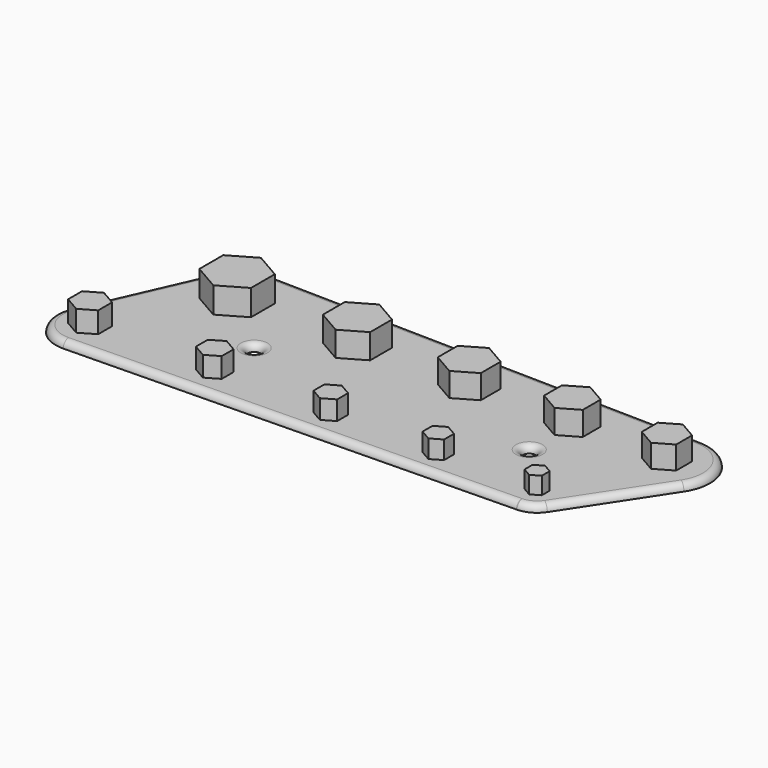
from build123d import *

# Parameters (mm, degrees)
F1_DEPTH  = 6.35
F2_DEPTH  = 3.175
F3_DEPTH  = 2.8222222222
F4_DEPTH  = 2.4694444444
F5_DEPTH  = 2.4694444444
F6_DEPTH  = 2.1166666667
F7_DEPTH  = 1.4111111111
F8_DEPTH  = 1.0583333333
F9_DEPTH  = 0.3527777778
F10_DEPTH = 0.7055555556
F12_DEPTH = 2.54
F13_R     = 2.38125
F14_DEPTH = 25.4
F15_R     = 2.53999
F16_R     = 2.53999
F18_DEPTH = 2.54


# Not quite as in the source:
# - a fillet or chamfer is up to 0.001 mm smaller than in the source, because OpenCascade refuses the exact size


with BuildPart() as f1:
    # F0 (on Top) → F1 (new body)
    with BuildSketch(Plane.XY):
        Polygon((152.4, 3.6661742094), (152.4, 0), (152.4, -3.6661742094), (158.75, -7.3323484187), (165.1, -3.6661742094), (165.1, 3.6661742094), (158.75, 7.3323484187), align=None)
    extrude(amount=F1_DEPTH)

    # F6 (add): a face of the model
    f6_faces = [f1.faces().sort_by_distance(p)[0] for p in [
        (158.75, 0, 6.35),
    ]]
    extrude(f6_faces, amount=F6_DEPTH)


with BuildPart() as f1b:
    # F0 (on Top) → F1, piece 2 (new body)
    with BuildSketch(Plane.XY):
        Polygon((144.4625, -36.2669128953), (141.2875, -34.4338257906), (138.1125, -36.2669128953), (138.1125, -39.9330871047), (141.2875, -41.7661742094), (144.4625, -39.9330871047), align=None)
    extrude(amount=F1_DEPTH)


with BuildPart() as f1c:
    # F0 (on Top) → F1, piece 3 (new body)
    with BuildSketch(Plane.XY):
        Polygon((116.68125, 4.1244459855), (116.68125, 0), (123.825, 0), (130.96875, 0), (130.96875, 4.1244459855), (123.825, 8.248891971), align=None)
        Polygon((123.825, 0), (116.68125, 0), (116.68125, -4.1244459855), (123.825, -8.248891971), (130.96875, -4.1244459855), (130.96875, 0), align=None)
    extrude(amount=F1_DEPTH)

    # F5 (add): a face of the model
    f5_faces = [f1c.faces().sort_by_distance(p)[0] for p in [
        (123.825, 0, 6.35),
    ]]
    extrude(f5_faces, amount=F5_DEPTH)


with BuildPart() as f1d:
    # F0 (on Top) → F1, piece 4 (new body)
    with BuildSketch(Plane.XY):
        Polygon((108.74375, -35.8086411192), (104.775, -33.5172822383), (100.80625, -35.8086411192), (100.80625, -40.3913588808), (104.775, -42.6827177617), (108.74375, -40.3913588808), align=None)
    extrude(amount=F1_DEPTH)

    # F9 (add): a face of the model
    f9_faces = [f1d.faces().sort_by_distance(p)[0] for p in [
        (104.775, -38.1, 6.35),
    ]]
    extrude(f9_faces, amount=F9_DEPTH)


with BuildPart() as f1e:
    # F0 (on Top) → F1, piece 5 (new body)
    with BuildSketch(Plane.XY):
        Polygon((77.7875, 4.5827177617), (77.7875, 0), (85.725, 0), (93.6625, 0), (93.6625, 4.5827177617), (85.725, 9.1654355234), align=None)
        Polygon((85.725, 0), (77.7875, 0), (77.7875, -4.5827177617), (85.725, -9.1654355234), (93.6625, -4.5827177617), (93.6625, 0), align=None)
    extrude(amount=F1_DEPTH)

    # F4 (add): a face of the model
    f4_faces = [f1e.faces().sort_by_distance(p)[0] for p in [
        (85.725, 0, 6.35),
    ]]
    extrude(f4_faces, amount=F4_DEPTH)


with BuildPart() as f1f:
    # F0 (on Top) → F1, piece 6 (new body)
    with BuildSketch(Plane.XY):
        Polygon((69.453125, -35.5795052311), (65.0875, -33.0590104621), (60.721875, -35.5795052311), (60.721875, -40.6204947689), (65.0875, -43.1409895379), (69.453125, -40.6204947689), align=None)
    extrude(amount=F1_DEPTH)

    # F10 (add): a face of the model
    f10_faces = [f1f.faces().sort_by_distance(p)[0] for p in [
        (65.0875, -38.1, 6.35),
    ]]
    extrude(f10_faces, amount=F10_DEPTH)


with BuildPart() as f1g:
    # F0 (on Top) → F1, piece 7 (new body)
    with BuildSketch(Plane.XY):
        Polygon((35.71875, 5.0409895379), (35.71875, 0), (44.45, 0), (53.18125, 0), (53.18125, 5.0409895379), (44.45, 10.0819790757), align=None)
        Polygon((44.45, 0), (35.71875, 0), (35.71875, -5.0409895379), (44.45, -10.0819790757), (53.18125, -5.0409895379), (53.18125, 0), align=None)
    extrude(amount=F1_DEPTH)

    # F3 (add): a face of the model
    f3_faces = [f1g.faces().sort_by_distance(p)[0] for p in [
        (44.45, 0, 6.35),
    ]]
    extrude(f3_faces, amount=F3_DEPTH)


with BuildPart() as f1h:
    # F0 (on Top) → F1, piece 8 (new body)
    with BuildSketch(Plane.XY):
        Polygon((-18.25625, -41.3079024332), (-18.25625, -38.1), (-18.25625, -34.8920975668), (-23.8125, -31.6841951336), (-29.36875, -34.8920975668), (-29.36875, -41.3079024332), (-23.8125, -44.5158048664), align=None)
    extrude(amount=F1_DEPTH)

    # F7 (add): a face of the model
    f7_faces = [f1h.faces().sort_by_distance(p)[0] for p in [
        (-23.8125, -38.1, 6.35),
    ]]
    extrude(f7_faces, amount=F7_DEPTH)


with BuildPart() as f1i:
    # F0 (on Top) → F1, piece 9 (new body)
    with BuildSketch(Plane.XY):
        Polygon((26.9875, -35.350369343), (22.225, -32.600738686), (22.225, -38.1), (17.4625, -38.1), (17.4625, -40.849630657), (22.225, -43.599261314), (26.9875, -40.849630657), align=None)
        Polygon((22.225, -38.1), (22.225, -32.600738686), (17.4625, -35.350369343), (17.4625, -38.1), align=None)
    extrude(amount=F1_DEPTH)

    # F8 (add): a face of the model
    f8_faces = [f1i.faces().sort_by_distance(p)[0] for p in [
        (22.225, -38.1, 6.35),
    ]]
    extrude(f8_faces, amount=F8_DEPTH)


with BuildPart() as f1j:
    # F0 (on Top) → F1, piece 10 (new body)
    with BuildSketch(Plane.XY):
        Polygon((9.525, -5.499261314), (9.525, 0), (9.525, 5.499261314), (0, 10.9985226281), (-9.525, 5.499261314), (-9.525, -5.499261314), (0, -10.9985226281), align=None)
    extrude(amount=F1_DEPTH)

    # F2 (add): a face of the model
    f2_faces = [f1j.faces().sort_by_distance(p)[0] for p in [
        (0, 0, 6.35),
    ]]
    extrude(f2_faces, amount=F2_DEPTH)


with BuildPart() as f12:
    # F11 (on face) → F12 (new body)
    with BuildSketch(Plane(origin=(0, 0, 0), x_dir=(1, 0, 0), z_dir=(0, 0, -1))):
        with BuildLine():
            Line((141.2875, 47.6267617683), (-23.5682692308, 50.7976514101))
            ThreePointArc((-23.5682692308, 50.7976514101), (-14.7463064556, 46.9934883266), (-11.1125, 38.1))
            Line((-11.1125, 38.1), (131.7625, 38.1))
            ThreePointArc((131.7625, 38.1), (134.617383755, 44.8996451583), (141.4706730769, 47.6232385575))
            Line((141.4706730769, 47.6232385575), (141.2875, 47.6267617683))
        make_face()
        with BuildLine():
            Line((-35.4252854215, 32.9586757782), (-17.4191781323, -7.7119863327))
            ThreePointArc((-17.4191781323, -7.7119863327), (-10.2318580693, -16.0689632662), (0.381, -19.0461896189))
            ThreePointArc((0.381, -19.0461896189), (13.6044211564, -13.335), (19.05, 0))
            Line((19.05, 0), (142.875, 0))
            ThreePointArc((142.875, 0), (147.6375, -11.3370176303), (159.0675, -15.8718246824))
            ThreePointArc((159.0675, -15.8718246824), (172.7981495603, -7.3935863375), (172.0126501051, 8.7245479648))
            Line((172.0126501051, 8.7245479648), (149.245090063, 43.3347287789))
            ThreePointArc((149.245090063, 43.3347287789), (145.8881342123, 46.4402511859), (141.4706730769, 47.6232385575))
            ThreePointArc((141.4706730769, 47.6232385575), (134.617383755, 44.8996451583), (131.7625, 38.1))
            Line((131.7625, 38.1), (-11.1125, 38.1))
            ThreePointArc((-11.1125, 38.1), (-14.7463064556, 46.9934883266), (-23.5682692308, 50.7976514101))
            ThreePointArc((-23.5682692308, 50.7976514101), (-34.3892798322, 45.1300589173), (-35.4252854215, 32.9586757782))
        make_face()
        Polygon((9.525, 5.499261314), (9.525, 0), (9.525, -5.499261314), (0, -10.9985226281), (-9.525, -5.499261314), (-9.525, 5.499261314), (0, 10.9985226281), align=None, mode=Mode.SUBTRACT)
        with BuildLine():
            ThreePointArc((19.05, 0), (13.6044211564, -13.335), (0.381, -19.0461896189))
            Line((0.381, -19.0461896189), (159.0675, -15.8718246824))
            ThreePointArc((159.0675, -15.8718246824), (147.6375, -11.3370176303), (142.875, 0))
            Line((142.875, 0), (19.05, 0))
        make_face()
    extrude(amount=F12_DEPTH)

    # F13 (on face) → F14 (cut)
    with BuildSketch(Plane(origin=(0, 0, -2.54), x_dir=(1, 0, 0), z_dir=(0, 0, -1))):
        with Locations((22.225, 19.900738686)):
            Circle(F13_R)
        with Locations((123.825, 19.900738686)):
            Circle(F13_R)
    extrude(amount=-F14_DEPTH, mode=Mode.SUBTRACT)

    # F15 (radius 2.54 in the source; OpenCascade refuses exactly that, so slightly less here)
    f15_edges = [f12.edges().sort_by_distance(p)[0] for p in [
        (19.84375, -19.900739, 0),
    ]]
    fillet(f15_edges, radius=F15_R)

    # F16 (radius 2.54 in the source; OpenCascade refuses exactly that, so slightly less here)
    f16_edges = [f12.edges().sort_by_distance(p)[0] for p in [
        (58.951202, -49.210445, 0),
        (121.44375, -19.900739, 0),
    ]]
    fillet(f16_edges, radius=F16_R)


with BuildPart() as f1j_1:
    add(f1j.part)

    # F17: union F1g, F1e, F1c, F1, F1h, F1i, F1f, F1d, F1b, F12
    add(f1g.part)
    add(f1e.part)
    add(f1c.part)
    add(f1.part)
    add(f1h.part)
    add(f1i.part)
    add(f1f.part)
    add(f1d.part)
    add(f1b.part)
    add(f12.part)

    # F18 (add, through all): a face of the model
    f18_faces = [f1j_1.faces().sort_by_distance(p)[0] for p in [
        (0, 0, 0),
    ]]
    extrude(f18_faces, amount=F18_DEPTH)


solid = f1j_1.part
